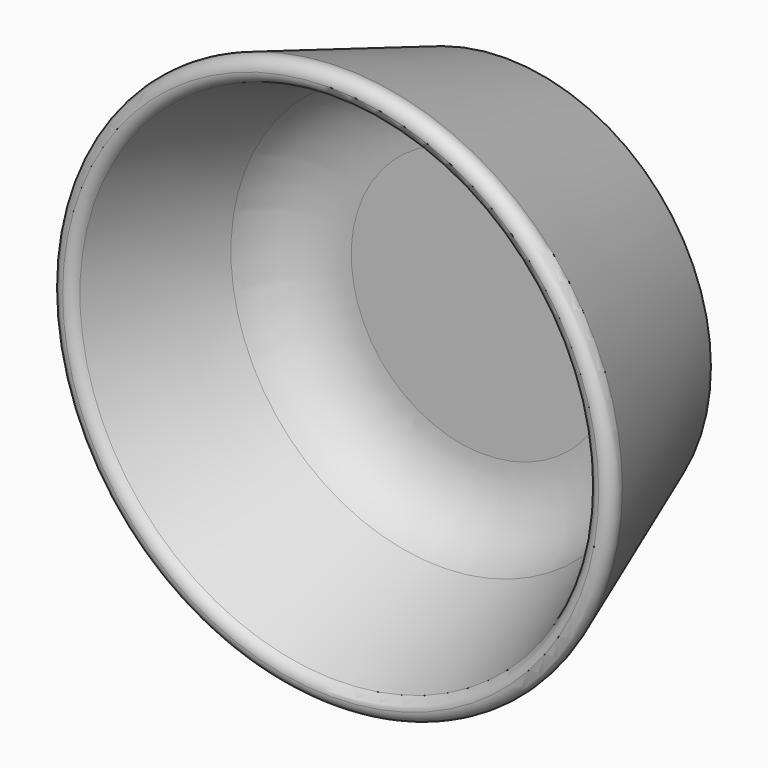
from build123d import *

# Parameters (mm, degrees)
F0_R     = 75
F1_DEPTH = 80
F1_TAPER = -20
F2_R     = 95
F3_DEPTH = 70
F3_TAPER = 20
F4_R     = 30
F5_R     = 4.283
F6_R     = 72.5
F7_DEPTH = 5


# Not quite as in the source:
# - a fillet or chamfer that OpenCascade refuses, or shapes differently, is made with other operations: its cross-section is extruded or revolved along the edge and cut away or added


with BuildPart() as f1:
    # F0 (on Front) → F1 (new body)
    with BuildSketch(Plane.XZ):
        Circle(F0_R)
    extrude(amount=F1_DEPTH, taper=F1_TAPER)

    # F2 (on face) → F3 (cut)
    with BuildSketch(Plane.XZ.offset(80)):
        Circle(F2_R)
    extrude(amount=-F3_DEPTH, taper=F3_TAPER, mode=Mode.SUBTRACT)

    # F4
    f4_edges = [f1.edges().sort_by_distance(p)[0] for p in [
        (-69.522084, -10, 0),
    ]]
    fillet(f4_edges, radius=F4_R)

    # F5
    f5_edges = [f1.edges().sort_by_distance(p)[0] for p in [
        (-95, -80, 0),
        (-104.117619, -80, 0),
    ]]
    fillet(f5_edges, radius=F5_R)

    # F6 (on face) → F7 (cut)
    with BuildSketch(Plane(origin=(0, 0, 0), x_dir=(-1, 0, 0), z_dir=(0, 1, 0))):
        Circle(F6_R)
    extrude(amount=-F7_DEPTH, mode=Mode.SUBTRACT)

    # F8: fillet of radius 7 on 1 edges, made by hand

    # F8_s1 → F8_t2 (revolve)
    with BuildSketch(Plane.XY):
        with BuildLine():
            ThreePointArc((-72.5, 0), (-69.9750962002, -3.6124860802), (-65.7917960675, -5))
            Line((-65.7917960675, -5), (-72.5, -5))
            Line((-72.5, -5), (-72.5, 0))
        make_face()
    revolve(axis=Axis((0, -5, 0), (0, 1, 0)))


solid = f1.part
